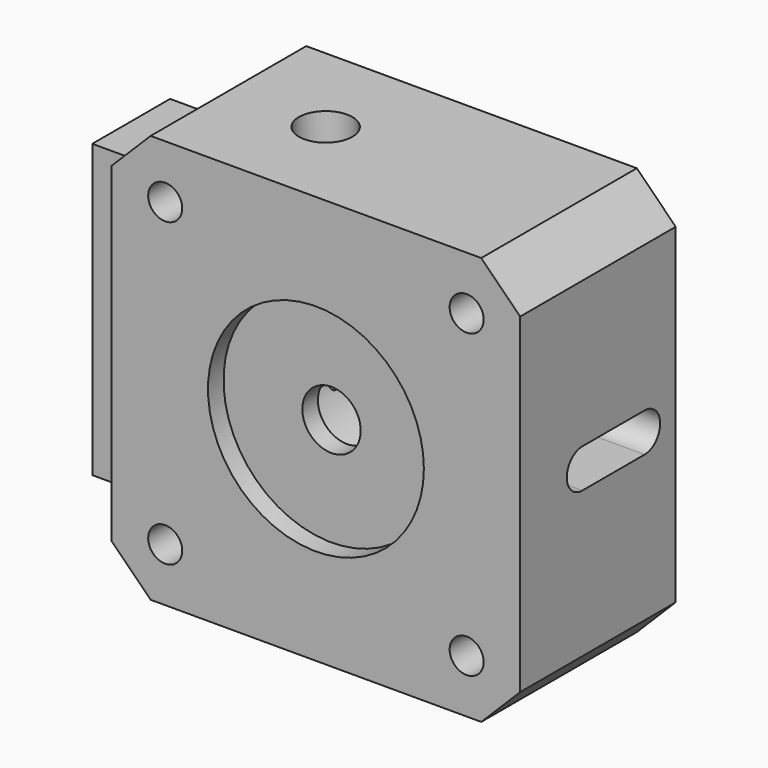
from build123d import *

# Parameters (mm, degrees)
F0_W      = 42
F0_H      = 42
F0_R      = 1.75
F0_R_2    = 3
F1_DEPTH  = 10
F2_R      = 11.1
F3_DEPTH  = 2
F4_R      = 1
F5_DEPTH  = 42
F7_DEPTH  = 16
F8_R      = 1.75
F9_DEPTH  = 12
F10_R     = 5
F10_R_2   = 1.5
F11_DEPTH = 2
F13_W     = 10
F13_H     = 30
F13_R     = 1.75
F14_DEPTH = 5
F15_W     = 2.75
F15_H     = 9
F16_DEPTH = 16
F18_DEPTH = 10
F19_R     = 2.75
F20_DEPTH = 5
F21_R     = 2.75
F22_DEPTH = 5
F23_R     = 1.35
F24_DEPTH = 10
F25_R     = 1.6
F26_DEPTH = 2.75
F27_SIZE  = 4
F28_W     = 2.5
F28_H     = 5.5
F29_DEPTH = 13.5
F31_REACH = 60.6501106407
F32_R     = 3
F33_DEPTH = 15


with BuildPart() as f1:
    # F0 (on Front) → F1 (new body, symmetric)
    with BuildSketch(Plane.XZ):
        Rectangle(F0_W, F0_H)
        with Locations((-15.5, -15.5)):
            Circle(F0_R, mode=Mode.SUBTRACT)
        with Locations((15.5, -15.5)):
            Circle(F0_R, mode=Mode.SUBTRACT)
        with Locations((-15.5, 15.5)):
            Circle(F0_R, mode=Mode.SUBTRACT)
        Circle(F0_R_2, mode=Mode.SUBTRACT)
        with Locations((15.5, 15.5)):
            Circle(F0_R, mode=Mode.SUBTRACT)
    extrude(amount=F1_DEPTH, both=True)

    # F2 (on face) → F3 (cut)
    with BuildSketch(Plane.XZ.offset(10)):
        Circle(F2_R)
    extrude(amount=-F3_DEPTH, mode=Mode.SUBTRACT)

    # F4 (on face) → F5 (cut, through all)
    with BuildSketch(Plane.XY.offset(21)):
        with Locations((-7, 0)):
            Circle(F4_R)
    extrude(amount=-F5_DEPTH, mode=Mode.SUBTRACT)

    # F6 (on face) → F7 (cut)
    with BuildSketch(Plane(origin=(0, 10, 0), x_dir=(-1, 0, 0), z_dir=(0, 1, 0))):
        with BuildLine():
            ThreePointArc((11.5, 5.5), (8.2705123017, 4.4520118156), (6.2717391304, 1.7074215296))
            ThreePointArc((6.2717391304, 1.7074215296), (-6.5, 0), (6.2717391304, -1.7074215296))
            ThreePointArc((6.2717391304, -1.7074215296), (8.2705123017, -4.4520118156), (11.5, -5.5))
            Line((11.5, -5.5), (21, -5.5))
            Line((21, -5.5), (21, 5.5))
            Line((21, 5.5), (11.5, 5.5))
        make_face()
    extrude(amount=-F7_DEPTH, mode=Mode.SUBTRACT)

    # F8 (on face) → F9 (cut)
    with BuildSketch(Plane(origin=(-21, 0, 0), x_dir=(0, -1, 0), z_dir=(-1, 0, 0))):
        with Locations((0, 10)):
            Circle(F8_R)
        with Locations((0, -10)):
            Circle(F8_R)
    extrude(amount=-F9_DEPTH, mode=Mode.SUBTRACT)

    # F19 (on face) → F20 (cut)
    with BuildSketch(Plane.XY.offset(21)):
        with Locations((-7, 0)):
            Circle(F19_R)
    extrude(amount=-F20_DEPTH, mode=Mode.SUBTRACT)

    # F21 (on face) → F22 (cut)
    with BuildSketch(Plane(origin=(0, 0, -21), x_dir=(1, 0, 0), z_dir=(0, 0, -1))):
        with Locations((-7, 0)):
            Circle(F21_R)
    extrude(amount=-F22_DEPTH, mode=Mode.SUBTRACT)

    # F27
    f27_edges = [f1.edges().sort_by_distance(p)[0] for p in [
        (21, 0, 21),
        (21, 0, -21),
        (-21, 0, -21),
        (-21, 0, 21),
    ]]
    chamfer(f27_edges, length=F27_SIZE)

    # F28 (on face) → F29 (cut)
    with BuildSketch(Plane(origin=(0, 10, 0), x_dir=(-1, 0, 0), z_dir=(0, 1, 0))):
        with Locations((18.25, 10)):
            Rectangle(F28_W, F28_H)
        with Locations((18.25, -10)):
            Rectangle(F28_W, F28_H)
    extrude(amount=-F29_DEPTH, mode=Mode.SUBTRACT)

    f31_end = f1.faces().sort_by_distance((6.5, 2, 0))[0]
    # F30 (on face) → F31 (cut, up to a face of the model that its end follows)
    with BuildSketch(Plane.YZ.offset(21)):
        with BuildLine():
            Line((6, 2), (-2, 2))
            ThreePointArc((-2, 2), (-4, 0), (-2, -2))
            Line((-2, -2), (6, -2))
            ThreePointArc((6, -2), (8, 0), (6, 2))
        make_face()
    f31_long = extrude(amount=-F31_REACH, mode=Mode.PRIVATE)
    add(split(f31_long, bisect_by=f31_end, keep=Keep.BOTTOM, mode=Mode.PRIVATE), mode=Mode.SUBTRACT)

    # F32 (on face) → F33 (cut)
    with BuildSketch(Plane(origin=(0, 10, 0), x_dir=(-1, 0, 0), z_dir=(0, 1, 0))):
        with Locations((-15.5, 15.5)):
            Circle(F32_R)
        with Locations((15.5, 15.5)):
            Circle(F32_R)
        with Locations((-15.5, -15.5)):
            Circle(F32_R)
        with Locations((15.5, -15.5)):
            Circle(F32_R)
    extrude(amount=-F33_DEPTH, mode=Mode.SUBTRACT)


with BuildPart() as f11:
    # F10 (on Front) → F11 (new body, symmetric)
    with BuildSketch(Plane.XZ):
        with Locations((-11.5, 0)):
            Circle(F10_R)
        with Locations((-11.5, 0)):
            Circle(F10_R_2, mode=Mode.SUBTRACT)
    extrude(amount=F11_DEPTH, both=True)


with BuildPart() as f14:
    # F13 (on offset) → F14 (new body)
    with BuildSketch(Plane(origin=(-22, 0, 0), x_dir=(0, -1, 0), z_dir=(-1, 0, 0))):
        Rectangle(F13_W, F13_H)
        with Locations((0, -10)):
            Circle(F13_R, mode=Mode.SUBTRACT)
        with Locations((0, 10)):
            Circle(F13_R, mode=Mode.SUBTRACT)
    extrude(amount=F14_DEPTH)

    # F15 (on face) → F16 (join)
    with BuildSketch(Plane.YZ.offset(-22)):
        with Locations((-3.625, 0)):
            Rectangle(F15_W, F15_H)
        with Locations((3.625, 0)):
            Rectangle(F15_W, F15_H)
    extrude(amount=F16_DEPTH)

    # F17 (on face) → F18 (cut, through all)
    with BuildSketch(Plane(origin=(0, 5, 0), x_dir=(-1, 0, 0), z_dir=(0, 1, 0))):
        with BuildLine():
            ThreePointArc((11.5, -4.5), (7, 0), (11.5, 4.5))
            Line((11.5, 4.5), (6, 4.5))
            Line((6, 4.5), (6, -4.5))
            Line((6, -4.5), (11.5, -4.5))
        make_face()
    extrude(amount=-F18_DEPTH, mode=Mode.SUBTRACT)

    # F23 (on face) → F24 (cut, through all)
    with BuildSketch(Plane(origin=(0, 5, 0), x_dir=(-1, 0, 0), z_dir=(0, 1, 0))):
        with Locations((11.5, 0)):
            Circle(F23_R)
    extrude(amount=-F24_DEPTH, mode=Mode.SUBTRACT)

    # F25 (on face) → F26 (cut, through all)
    with BuildSketch(Plane(origin=(0, 5, 0), x_dir=(-1, 0, 0), z_dir=(0, 1, 0))):
        with Locations((11.5, 0)):
            Circle(F25_R)
    extrude(amount=-F26_DEPTH, mode=Mode.SUBTRACT)


solid = Compound([f1.part, f11.part, f14.part])
